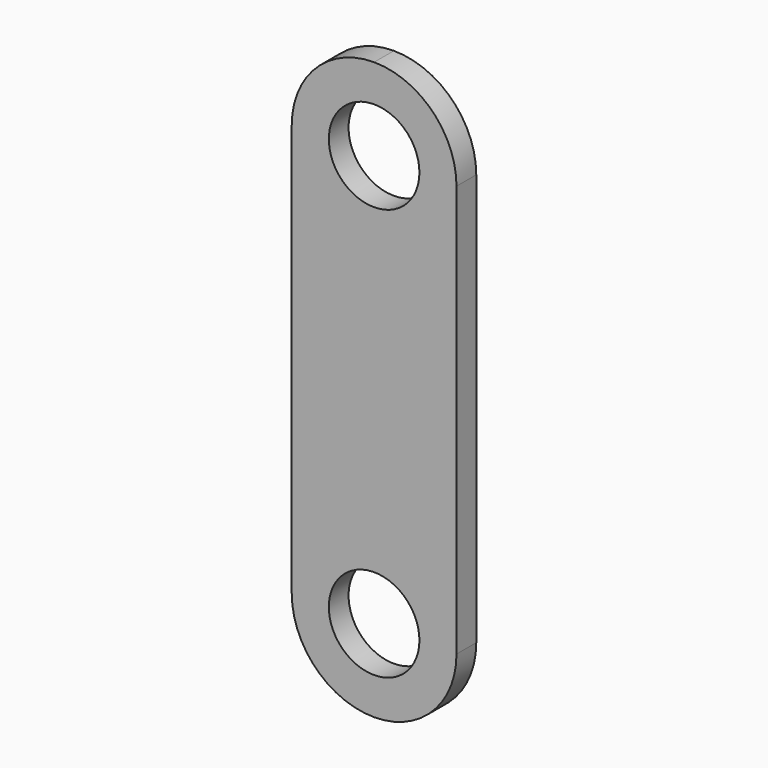
from build123d import *

# Parameters (mm, degrees)
F0_W     = 40
F0_H     = 140
F0_R     = 11
F1_DEPTH = 6
F2_R     = 19.99999


# Not quite as in the source:
# - a fillet or chamfer is up to 0.001 mm smaller than in the source, because OpenCascade refuses the exact size


with BuildPart() as f1:
    # F0 (on Front) → F1 (new body)
    with BuildSketch(Plane.XZ):
        with Locations((0, -50)):
            Rectangle(F0_W, F0_H)
        with Locations((0, -100)):
            Circle(F0_R, mode=Mode.SUBTRACT)
        Circle(F0_R, mode=Mode.SUBTRACT)
    extrude(amount=F1_DEPTH)

    # F2 (radius 20 in the source; OpenCascade refuses exactly that, so slightly less here)
    f2_edges = [f1.edges().sort_by_distance(p)[0] for p in [
        (20, -3, 20),
        (-20, -3, 20),
        (-20, -3, -120),
        (20, -3, -120),
    ]]
    fillet(f2_edges, radius=F2_R)


solid = f1.part
